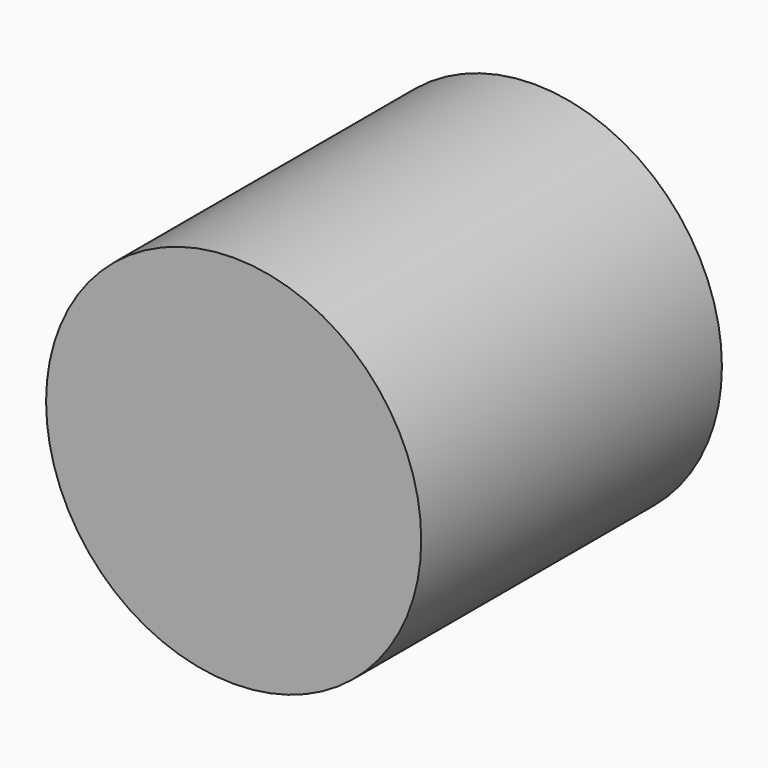
from build123d import *

# Parameters (mm, degrees)
F2_R     = 63.3866016578
F3_DEPTH = 127


# Not quite as in the source:
# - the program builds the solid bodies; features that only make, move or delete a surface that nothing else refers to are left out


with BuildPart() as f3:
    # F2 (on face) → F3 (new body)
    with BuildSketch(Plane.XZ):
        Circle(F2_R)
    extrude(amount=F3_DEPTH)


solid = f3.part
